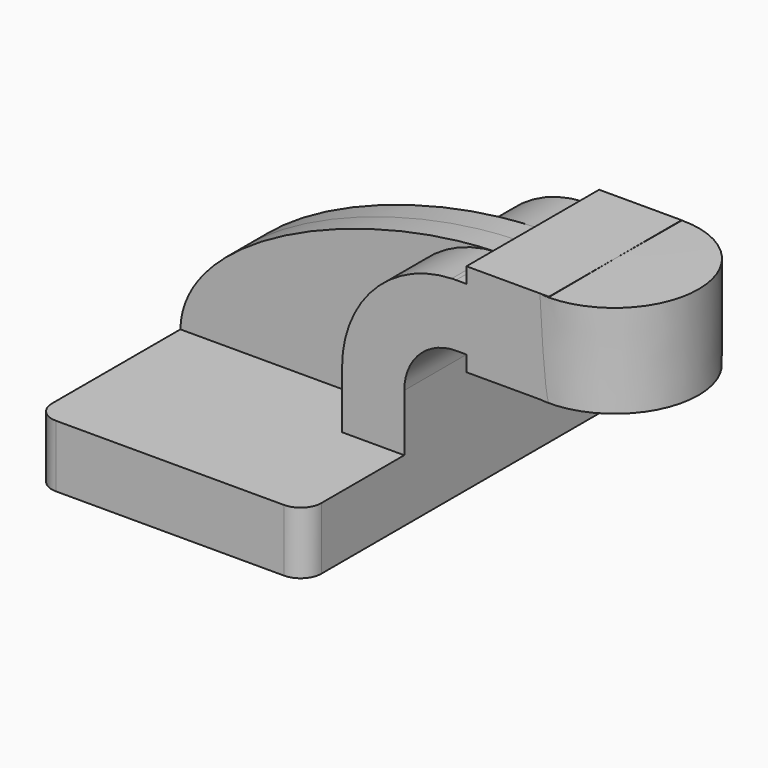
from build123d import *

# Parameters (mm, degrees)
F1_DEPTH = 63.5
F2_DEPTH = 25.4
F3_DEPTH = 7.9375
F5_R     = 6.35


with BuildPart() as f1:
    # F0 (on Front) → F1 (new body, symmetric)
    with BuildSketch(Plane.XZ):
        Polygon((-41.275, 9.525), (-41.275, -9.525), (41.275, -9.525), (41.275, 9.525), (22.225, 9.525), align=None)
    extrude(amount=F1_DEPTH, both=True)

    # F0 (on Front) → F2 (join, symmetric)
    with BuildSketch(Plane.XZ):
        with BuildLine():
            Line((22.225, 9.525), (41.275, 9.525))
            Line((41.275, 9.525), (41.275, 27.0002))
            ThreePointArc((41.275, 27.0002), (45.9246798487, 38.2255201513), (57.15, 42.8752))
            Line((57.15, 42.8752), (60.325, 42.8752))
            Line((60.325, 42.8752), (60.325, 61.9252))
            Line((60.325, 61.9252), (57.15, 61.9252))
            add(Edge.make_bspline(
                [(55.8342690967, 61.900407409), (56.274218932, 61.9111436169), (56.7128210879, 61.9194148517), (57.15, 61.9252)],
                knots=[110.352429098, 110.352429098, 110.352429098, 110.352429098, 111.5045361635, 111.5045361635, 111.5045361635, 111.5045361635], degree=3))
            ThreePointArc((55.8342690967, 61.900407409), (31.9934151086, 51.2262574919), (22.225, 27.0002))
            Line((22.225, 27.0002), (22.225, 9.525))
        make_face()
        Polygon((60.325, 66.675), (60.325, 61.9252), (60.325, 42.8752), (60.325, 38.1), (85.725, 38.1), (85.576608777, 66.675), align=None)
    extrude(amount=F2_DEPTH, both=True)

    # F0 (on Front) → F3 (join, symmetric)
    with BuildSketch(Plane.XZ):
        with BuildLine():
            add(Edge.make_bspline(
                [(-41.275, 9.525), (-40.8094440998, 37.2290406247), (13.6944936723, 60.8720597372), (55.8342690967, 61.900407409)],
                knots=[0, 0, 0, 0, 110.352429098, 110.352429098, 110.352429098, 110.352429098], degree=3))
            Line((-41.275, 9.525), (22.225, 9.525))
            Line((22.225, 9.525), (22.225, 27.0002))
            ThreePointArc((22.225, 27.0002), (31.9934151086, 51.2262574919), (55.8342690967, 61.900407409))
        make_face()
    extrude(amount=F3_DEPTH, both=True)

    # F0 (on Front) → F4 (revolve)
    with BuildSketch(Plane.XZ):
        Polygon((111.125, 66.675), (85.576608777, 66.675), (85.725, 38.1), (111.125, 38.1), align=None)
    revolve(axis=Axis((85.6508043885, 0, 52.3875), (-0.0051929737, 0, 0.9999865164)))

    # F5
    f5_edges = [f1.edges().sort_by_distance(p)[0] for p in [
        (-41.275, -63.5, 0),
        (41.275, -63.5, 0),
        (41.275, 63.5, 0),
        (-41.275, 63.5, 0),
    ]]
    fillet(f5_edges, radius=F5_R)


solid = f1.part
